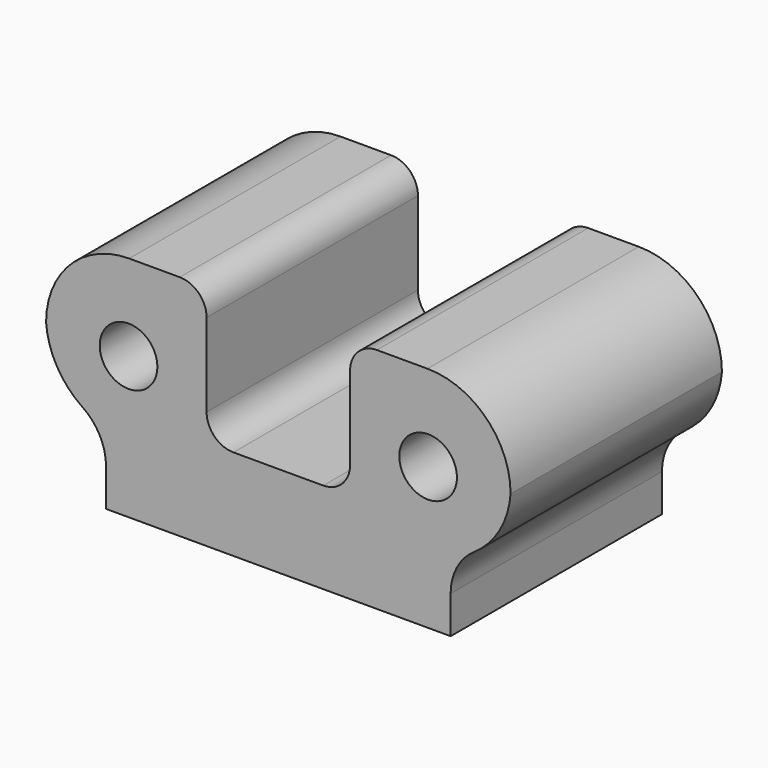
from build123d import *

# Parameters (mm, degrees)
F0_R        = 2.7305
F1_DEPTH    = 25.019
F2_R        = 2.54
F3_R        = 7.874
F4_R        = 5.08
F5_T1_DEPTH = 50.419


# Not quite as in the source:
# - a fillet or chamfer that OpenCascade refuses, or shapes differently, is made with other operations: its cross-section is extruded or revolved along the edge and cut away or added


with BuildPart() as f1:
    # F0 (on Front) → F1 (new body)
    with BuildSketch(Plane.XZ):
        Polygon((-6.7945, 10.795), (-21.9964, 10.795), (-21.9964, -2.159), (-16.3195, -2.159), (-16.3195, -10.795), (0, -10.795), (16.3195, -10.795), (16.3195, -2.159), (21.9964, -2.159), (21.9964, 10.795), (6.7945, 10.795), (6.7945, -2.159), (0, -2.159), (-6.7945, -2.159), align=None)
        with Locations((-14.1859, 2.6289)):
            Circle(F0_R, mode=Mode.SUBTRACT)
        with Locations((14.1859, 2.6289)):
            Circle(F0_R, mode=Mode.SUBTRACT)
    extrude(amount=F1_DEPTH)

    # F2
    f2_edges = [f1.edges().sort_by_distance(p)[0] for p in [
        (-6.7945, -12.5095, 10.795),
        (-6.7945, -12.5095, -2.159),
        (6.7945, -12.5095, -2.159),
        (6.7945, -12.5095, 10.795),
    ]]
    fillet(f2_edges, radius=F2_R)

    # F3
    f3_edges = [f1.edges().sort_by_distance(p)[0] for p in [
        (-21.9964, -12.5095, 10.795),
        (21.9964, -12.5095, 10.795),
    ]]
    fillet(f3_edges, radius=F3_R)

    # F4
    f4_edges = [f1.edges().sort_by_distance(p)[0] for p in [
        (-16.3195, -12.5095, -2.159),
        (16.3195, -12.5095, -2.159),
    ]]
    fillet(f4_edges, radius=F4_R)

    # F5: fillet of radius 7.874 on 2 edges, made by hand

    # F5_s2 → F5_t1 (cut)
    with BuildSketch(Plane.XZ.offset(-12.7)):
        with BuildLine():
            ThreePointArc((-18.5538606902, -3.0308249896), (-20.9591016403, -0.4505219212), (-21.9964, 2.921))
            Line((-21.9964, 2.921), (-22.781728024, 2.8639153723))
            ThreePointArc((-22.781728024, 2.8639153723), (-22.7838, 0.381), (-22.7838, -2.159))
            Line((-22.7838, -2.159), (-21.9964, -2.9464))
            ThreePointArc((-21.9964, -2.9464), (-21.3995, -2.9464), (-18.9949347832, -3.6830921162))
            Line((-18.9949347832, -3.6830921162), (-18.5538606902, -3.0308249896))
        make_face()
        with BuildLine():
            ThreePointArc((18.5538606902, -3.0308249896), (20.9591016403, -0.4505219212), (21.9964, 2.921))
            Line((21.9964, 2.921), (22.781728024, 2.8639153723))
            ThreePointArc((22.781728024, 2.8639153723), (22.7838, 0.381), (22.7838, -2.159))
            Line((22.7838, -2.159), (21.9964, -2.9464))
            ThreePointArc((21.9964, -2.9464), (21.3995, -2.9464), (18.9949347832, -3.6830921162))
            Line((18.9949347832, -3.6830921162), (18.5538606902, -3.0308249896))
        make_face()
    extrude(amount=F5_T1_DEPTH, mode=Mode.SUBTRACT)


solid = f1.part
